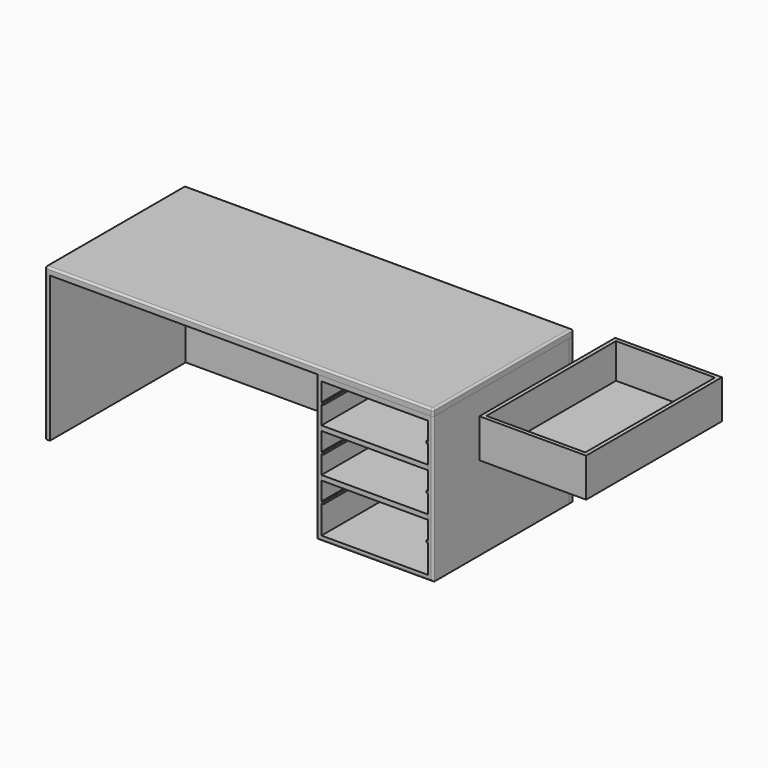
from build123d import *

# Parameters (mm, degrees)
F0_W           = 2000
F0_H           = 900
F1_DEPTH       = 35
F2_R           = 10
F3_W           = 600
F3_H           = 750
F3_W_2         = 550
F3_H_2         = 700
F4_DEPTH       = 875
F5_R           = 10
F6_W           = 900
F6_H           = 750
F7_DEPTH       = 25
F8_W           = 1975
F8_H           = 750
F9_DEPTH       = 25
F10_T1_DEPTH   = 50
F10_S5_W       = 10
F10_S5_H       = 10
F10_T6_DEPTH   = 10
F10_2_T1_DEPTH = 800
F11_T1_DEPTH   = 50
F11_S5_W       = 10
F11_S5_H       = 10
F11_T6_DEPTH   = 10
F12_W          = 550
F12_H          = 25
F13_DEPTH      = 875
F14_W          = 550
F14_H          = 25
F15_DEPTH      = 875
F16_W          = 875
F16_H          = 10
F17_DEPTH      = 10
F18_W          = 875
F18_H          = 10
F19_DEPTH      = 10
F20_W          = 550
F20_H          = 875
F21_DEPTH      = 200
F22_T          = -20


# Not quite as in the source:
# - a fillet or chamfer that OpenCascade refuses, or shapes differently, is made with other operations: its cross-section is extruded or revolved along the edge and cut away or added


with BuildPart() as f1:
    # F0 (on Top) → F1 (new body)
    with BuildSketch(Plane.XY):
        with Locations((-1000, 450)):
            Rectangle(F0_W, F0_H)
    extrude(amount=F1_DEPTH)

    # F2
    f2_edges = [f1.edges().sort_by_distance(p)[0] for p in [
        (-2000, 450, 35),
        (-1000, 900, 35),
        (0, 450, 35),
        (-1000, 0, 35),
    ]]
    fillet(f2_edges, radius=F2_R)

    # F10: fillet of radius 10 on 1 edges, made by hand

    # F10_s2 → F10_t1 (cut)
    with BuildSketch(Plane.XY.offset(-25)):
        with BuildLine():
            ThreePointArc((-1990, 0), (-1997.0710678119, 2.9289321881), (-2000, 10))
            Line((-2000, 10), (-2000, 0))
            Line((-2000, 0), (-1990, 0))
        make_face()
    extrude(amount=F10_T1_DEPTH, mode=Mode.SUBTRACT)


with BuildPart() as f4:
    # F3 (on Front) → F4 (new body)
    with BuildSketch(Plane.XZ):
        with Locations((-300, -375)):
            Rectangle(F3_W, F3_H)
        with Locations((-300, -375)):
            Rectangle(F3_W_2, F3_H_2, mode=Mode.SUBTRACT)
    extrude(amount=-F4_DEPTH)

    # F5
    f5_edges = [f4.edges().sort_by_distance(p)[0] for p in [
        (-600, 0, -375),
        (-300, 0, -750),
        (0, 0, -375),
    ]]
    fillet(f5_edges, radius=F5_R)


with BuildPart() as f7:
    # F6 (on face) → F7 (new body)
    with BuildSketch(Plane(origin=(-2000, 0, 0), x_dir=(0, -1, 0), z_dir=(-1, 0, 0))):
        with Locations((-450, -375)):
            Rectangle(F6_W, F6_H)
    extrude(amount=-F7_DEPTH)

    # F10#2: fillet of radius 10 on 1 edges, made by hand

    # F10_2_s2 → F10_2_t1 (cut)
    with BuildSketch(Plane.XY.offset(-775)):
        with BuildLine():
            ThreePointArc((-1990, 0), (-1997.0710678119, 2.9289321881), (-2000, 10))
            Line((-2000, 10), (-2000, 0))
            Line((-2000, 0), (-1990, 0))
        make_face()
    extrude(amount=F10_2_T1_DEPTH, mode=Mode.SUBTRACT)


with BuildPart() as f9:
    # F8 (on face) → F9 (new body)
    with BuildSketch(Plane(origin=(0, 900, 0), x_dir=(-1, 0, 0), z_dir=(0, 1, 0))):
        with Locations((987.5, -375)):
            Rectangle(F8_W, F8_H)
    extrude(amount=-F9_DEPTH)


with BuildPart() as f10_tool4:
    # F10_s5 → F10_t6 (new body)
    with BuildSketch(Plane.XZ.offset(-10)):
        with Locations((-1995, 30)):
            Rectangle(F10_S5_W, F10_S5_H)
    extrude(amount=F10_T6_DEPTH)

    # F10_s7 → F10_t8 (revolve, cut)
    with BuildSketch(Plane(origin=(-1990, 10, 25), x_dir=(0.7071067812, 0, -0.7071067812), z_dir=(-0.7071067812, 0, -0.7071067812))):
        with BuildLine():
            ThreePointArc((0, -10), (10, 0), (0, 10))
            Line((0, 10), (0, -10))
        make_face()
    revolve(axis=Axis((-1990, 10, 25), (0, -1, 0)), mode=Mode.SUBTRACT)


with BuildPart() as f1_1:
    add(f1.part)

    # F10_t3: cut F10_tool4
    add(f10_tool4.part, mode=Mode.SUBTRACT)

    # F11: fillet of radius 10 on 1 edges, made by hand

    # F11_s2 → F11_t1 (cut)
    with BuildSketch(Plane.XY.offset(-25)):
        with BuildLine():
            ThreePointArc((-10, 0), (-2.9289321881, 2.9289321881), (0, 10))
            Line((0, 10), (0, 0))
            Line((0, 0), (-10, 0))
        make_face()
    extrude(amount=F11_T1_DEPTH, mode=Mode.SUBTRACT)


with BuildPart() as f11_tool4:
    # F11_s5 → F11_t6 (new body)
    with BuildSketch(Plane.XZ.offset(-10)):
        with Locations((-5, 30)):
            Rectangle(F11_S5_W, F11_S5_H)
    extrude(amount=F11_T6_DEPTH)

    # F11_s7 → F11_t8 (revolve, cut)
    with BuildSketch(Plane(origin=(-10, 10, 25), x_dir=(-0.7071067812, 0, -0.7071067812), z_dir=(-0.7071067812, 0, 0.7071067812))):
        with BuildLine():
            ThreePointArc((0, -10), (10, 0), (0, 10))
            Line((0, 10), (0, -10))
        make_face()
    revolve(axis=Axis((-10, 10, 25), (0, -1, 0)), mode=Mode.SUBTRACT)


with BuildPart() as f1_2:
    add(f1_1.part)

    # F11_t3: cut F11_tool4
    add(f11_tool4.part, mode=Mode.SUBTRACT)


with BuildPart() as f13:
    # F12 (on face) → F13 (new body)
    with BuildSketch(Plane.XZ):
        with Locations((-300, -237.5)):
            Rectangle(F12_W, F12_H)
    extrude(amount=-F13_DEPTH)


with BuildPart() as f15:
    # F14 (on face) → F15 (new body)
    with BuildSketch(Plane.XZ):
        with Locations((-300, -462.5)):
            Rectangle(F14_W, F14_H)
    extrude(amount=-F15_DEPTH)


with BuildPart() as f17:
    # F16 (on face) → F17 (new body)
    with BuildSketch(Plane.YZ.offset(-575)):
        with Locations((437.5, -125)):
            Rectangle(F16_W, F16_H)
    extrude(amount=F17_DEPTH)


with BuildPart() as f17b:
    # F16 (on face) → F17, piece 2 (new body)
    with BuildSketch(Plane.YZ.offset(-575)):
        with Locations((437.5, -350)):
            Rectangle(F16_W, F16_H)
    extrude(amount=F17_DEPTH)


with BuildPart() as f17c:
    # F16 (on face) → F17, piece 3 (new body)
    with BuildSketch(Plane.YZ.offset(-575)):
        with Locations((437.5, -575)):
            Rectangle(F16_W, F16_H)
    extrude(amount=F17_DEPTH)


with BuildPart() as f19:
    # F18 (on face) → F19 (new body)
    with BuildSketch(Plane(origin=(-25, 0, 0), x_dir=(0, -1, 0), z_dir=(-1, 0, 0))):
        with Locations((-437.5, -125)):
            Rectangle(F18_W, F18_H)
    extrude(amount=F19_DEPTH)


with BuildPart() as f19b:
    # F18 (on face) → F19, piece 2 (new body)
    with BuildSketch(Plane(origin=(-25, 0, 0), x_dir=(0, -1, 0), z_dir=(-1, 0, 0))):
        with Locations((-437.5, -350)):
            Rectangle(F18_W, F18_H)
    extrude(amount=F19_DEPTH)


with BuildPart() as f19c:
    # F18 (on face) → F19, piece 3 (new body)
    with BuildSketch(Plane(origin=(-25, 0, 0), x_dir=(0, -1, 0), z_dir=(-1, 0, 0))):
        with Locations((-437.5, -575)):
            Rectangle(F18_W, F18_H)
    extrude(amount=F19_DEPTH)


with BuildPart() as f21:
    # F20 (on face) → F21 (new body)
    with BuildSketch(Plane.XY.offset(35)):
        with Locations((458.4253653884, 507.1054147508)):
            Rectangle(F20_W, F20_H)
    extrude(amount=-F21_DEPTH)

    # F22
    f22_openings = [f21.faces().sort_by_distance(p)[0] for p in [
        (458.425365, 507.105415, 35),
    ]]
    offset(amount=F22_T, openings=f22_openings)


solid = Compound([f4.part, f7.part, f9.part, f1_2.part, f13.part, f15.part, f17.part, f17b.part, f17c.part, f19.part, f19b.part, f19c.part, f21.part])
